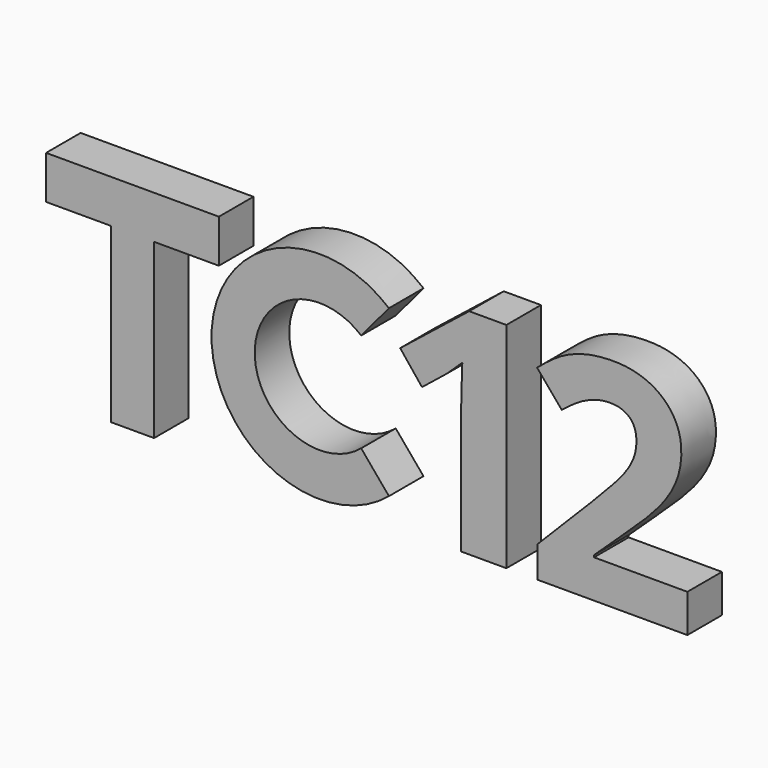
from build123d import *

# Parameters (mm, degrees)
F0_W         = 25.4
F0_H         = 101.6
F0_TEXT_SIZE = 176.3888888889
F1_DEPTH     = 25.4


# Not quite as in the source:
# - Text() gives the source's letters only with a copy of the font that has no kerning and outlines rounded to 1/6400 em; it was checked with that copy


with BuildPart() as f1:
    # F0 (on Front) → F1 (new body)
    with BuildSketch(Plane.XZ):
        Polygon((-45.2788638287, 127), (-146.8788638287, 127), (-146.8788638287, 101.6), (-108.7788638287, 101.6), (-83.3788638287, 101.6), (-45.2788638287, 101.6), align=None)
        with Locations((-96.0788638287, 50.8)):
            Rectangle(F0_W, F0_H)
        with BuildLine():
            Line((38.3916385767, 92.6862932828), (54.7184438628, 112.1438221381))
            ThreePointArc((54.7184438628, 112.1438221381), (-49.5985693523, 63.5), (54.7184438628, 14.8561778619))
            Line((54.7184438628, 14.8561778619), (38.3916385767, 34.3137067172))
            ThreePointArc((38.3916385767, 34.3137067172), (-24.1985693523, 63.5), (38.3916385767, 92.6862932828))
        make_face()
        with Locations((50.90117082, 0)):
            Text('1', F0_TEXT_SIZE, font='Open Sans', font_style=FontStyle.BOLD, text_align=(TextAlign.LEFT, TextAlign.BOTTOM))
        with Locations((135.09722054, 0)):
            Text('2', F0_TEXT_SIZE, font='Open Sans', font_style=FontStyle.BOLD, text_align=(TextAlign.LEFT, TextAlign.BOTTOM))
    extrude(amount=F1_DEPTH)


solid = f1.part
